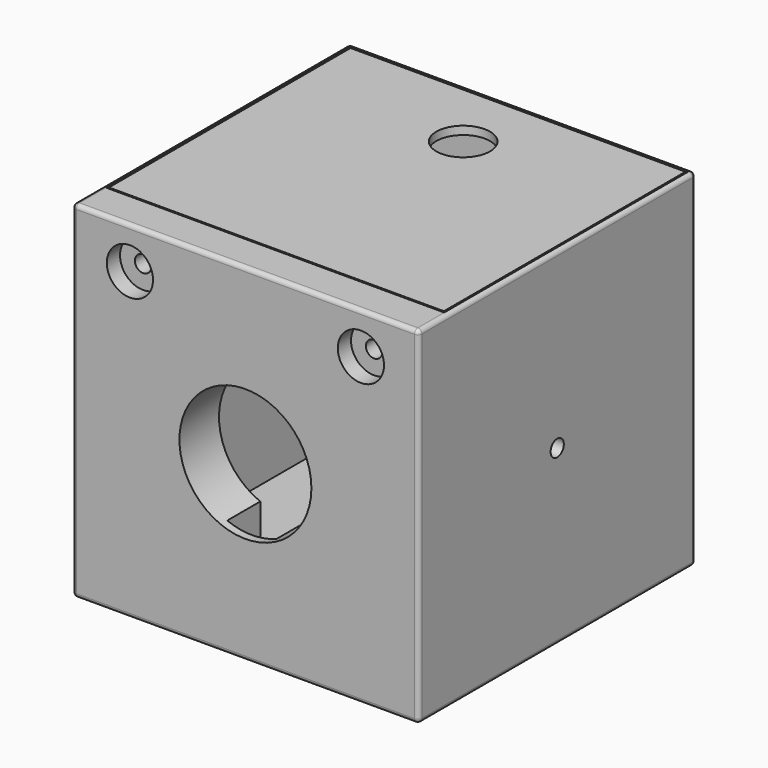
from build123d import *

# Parameters (mm, degrees)
F0_W      = 42
F0_H      = 42
F1_DEPTH  = 42
F2_T      = -2
F3_R      = 8
F4_DEPTH  = 21.001
F5_DEPTH  = 4
F7_W      = 6
F7_H      = 5
F8_DEPTH  = 5.5848015129
F9_R      = 3.85
F10_DEPTH = 2
F11_W     = 41
F11_H     = 37
F12_DEPTH = 1
F13_W     = 40.6
F13_H     = 36.6
F14_DEPTH = 1
F15_W     = 22
F15_H     = 3
F16_DEPTH = 35
F17_W     = 37
F17_H     = 3
F18_DEPTH = 2.5
F19_W     = 9
F19_H     = 3
F20_DEPTH = 15
F21_R     = 1
F22_DEPTH = 10
F23_R     = 1
F24_DEPTH = 25
F25_R     = 2.8
F26_DEPTH = 2
F27_R     = 1
F28_DEPTH = 42.001
F29_R     = 3.25
F30_DEPTH = 1
F31_R     = 0.49999


# Not quite as in the source:
# - a fillet or chamfer is up to 0.001 mm smaller than in the source, because OpenCascade refuses the exact size


with BuildPart() as f1:
    # F0 (on Top) → F1 (new body)
    with BuildSketch(Plane.XY):
        Rectangle(F0_W, F0_H)
    extrude(amount=F1_DEPTH)

    # F2
    f2_openings = [f1.faces().sort_by_distance(p)[0] for p in [
        (0, 0, 42),
    ]]
    offset(amount=F2_T, openings=f2_openings)

    # F3 (on Front) → F4 (cut, through all)
    with BuildSketch(Plane.XZ):
        with Locations((0, 21)):
            Circle(F3_R)
    extrude(amount=F4_DEPTH, mode=Mode.SUBTRACT)

    # F5 (add): a face of the model
    f5_faces = [f1.faces().sort_by_distance(p)[0] for p in [
        (0, -19, 41.448275431),
    ]]
    extrude(f5_faces, amount=F5_DEPTH)

    # F7 (on offset) → F8 (cut, through all)
    with BuildSketch(Plane.XY.offset(8)):
        with Locations((0, -17.5)):
            Rectangle(F7_W, F7_H)
    extrude(amount=F8_DEPTH, mode=Mode.SUBTRACT)

    # F9 (on face) → F10 (cut, through all)
    with BuildSketch(Plane(origin=(0, 21, 0), x_dir=(-1, 0, 0), z_dir=(0, 1, 0))):
        with Locations((-11, 20)):
            Circle(F9_R)
    extrude(amount=-F10_DEPTH, mode=Mode.SUBTRACT)

    # F11 (on face) → F12 (cut)
    with BuildSketch(Plane.XY.offset(42)):
        with Locations((0, 2)):
            Rectangle(F11_W, F11_H)
    extrude(amount=-F12_DEPTH, mode=Mode.SUBTRACT)


with BuildPart() as f14:
    # F13 (on face) → F14 (new body, through all)
    with BuildSketch(Plane.XY.offset(41)):
        with Locations((0, 2)):
            Rectangle(F13_W, F13_H)
    extrude(amount=F14_DEPTH)

    # F15 (on face) → F16 (join)
    with BuildSketch(Plane(origin=(0, 0, 41), x_dir=(1, 0, 0), z_dir=(0, 0, -1))):
        with Locations((-7.5, -17)):
            Rectangle(F15_W, F15_H)
    extrude(amount=F16_DEPTH)

    # F17 (on face) → F18 (join)
    with BuildSketch(Plane(origin=(0, 0, 41), x_dir=(1, 0, 0), z_dir=(0, 0, -1))):
        with Locations((0, 13)):
            Rectangle(F17_W, F17_H)
    extrude(amount=F18_DEPTH)

    # F19 (on face) → F20 (join)
    with BuildSketch(Plane(origin=(0, 0, 38.5), x_dir=(1, 0, 0), z_dir=(0, 0, -1))):
        with Locations((14, 13)):
            Rectangle(F19_W, F19_H)
        with Locations((-14, 13)):
            Rectangle(F19_W, F19_H)
    extrude(amount=F20_DEPTH)


with BuildPart() as f22_tool:
    # F21 (on face) → F22 (new body)
    with BuildSketch(Plane(origin=(0, 21, 0), x_dir=(-1, 0, 0), z_dir=(0, 1, 0))):
        with Locations((0, 37)):
            Circle(F21_R)
    extrude(amount=-F22_DEPTH)


with BuildPart() as f1_1:
    add(f1.part)

    # F22: cut by f22_tool
    add(f22_tool.part, mode=Mode.SUBTRACT)


with BuildPart() as f14_1:
    add(f14.part)

    # F22: cut by f22_tool
    add(f22_tool.part, mode=Mode.SUBTRACT)


with BuildPart() as f24_tool:
    # F23 (on face) → F24 (new body)
    with BuildSketch(Plane.XZ.offset(21)):
        with Locations((-14, 37)):
            Circle(F23_R)
        with Locations((14, 37)):
            Circle(F23_R)
    extrude(amount=-F24_DEPTH)


with BuildPart() as f1_2:
    add(f1_1.part)

    # F24: cut by f24_tool
    add(f24_tool.part, mode=Mode.SUBTRACT)

    # F25 (on face) → F26 (cut)
    with BuildSketch(Plane.XZ.offset(21)):
        with Locations((14, 37)):
            Circle(F25_R)
        with Locations((-14, 37)):
            Circle(F25_R)
    extrude(amount=-F26_DEPTH, mode=Mode.SUBTRACT)

    # F27 (on face) → F28 (cut, through all)
    with BuildSketch(Plane.YZ.offset(21)):
        with Locations((0, 21)):
            Circle(F27_R)
    extrude(amount=-F28_DEPTH, mode=Mode.SUBTRACT)

    # F31 (radius 0.5 in the source; OpenCascade refuses exactly that, so slightly less here)
    f31_edges = [f1_2.edges().sort_by_distance(p)[0] for p in [
        (21, 0, 42),
        (0, 21, 42),
        (21, 21, 21),
        (-21, 21, 21),
        (0, 21, 0),
        (21, 0, 0),
        (21, -21, 21),
        (0, -21, 42),
        (-21, 0, 42),
        (-21, -21, 21),
        (-21, 0, 0),
        (0, -21, 0),
    ]]
    fillet(f31_edges, radius=F31_R)


with BuildPart() as f14_2:
    add(f14_1.part)

    # F24: cut by f24_tool
    add(f24_tool.part, mode=Mode.SUBTRACT)

    # F29 (on face) → F30 (cut, through all)
    with BuildSketch(Plane.XY.offset(42)):
        with Locations((0, 12)):
            Circle(F29_R)
    extrude(amount=-F30_DEPTH, mode=Mode.SUBTRACT)


solid = Compound([f1_2.part, f14_2.part])
